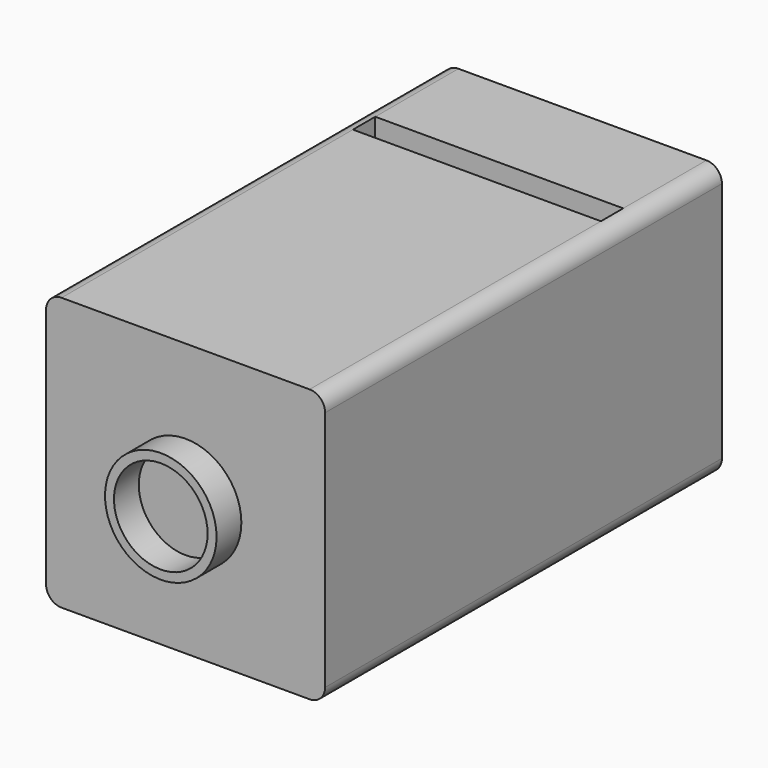
from build123d import *

# Parameters (mm, degrees)
F0_W     = 90
F0_H     = 160
F1_DEPTH = 88
F2_W     = 80
F2_H     = 9
F3_DEPTH = 12.5
F4_DEPTH = 50
F5_R     = 17.988747928
F6_DEPTH = 10
F7_R     = 15.1004844519
F8_DEPTH = 10
F9_R     = 4.99999


# Not quite as in the source:
# - a fillet or chamfer is up to 0.001 mm smaller than in the source, because OpenCascade refuses the exact size


with BuildPart() as f1:
    # F0 (on Top) → F1 (new body)
    with BuildSketch(Plane.XY):
        Rectangle(F0_W, F0_H)
    extrude(amount=F1_DEPTH)

    # F2 (on face) → F3 (cut, symmetric)
    with BuildSketch(Plane.XY.offset(88)):
        with Locations((0, 41.9618518679)):
            Rectangle(F2_W, F2_H)
    extrude(amount=F3_DEPTH, both=True, mode=Mode.SUBTRACT)

    # F4 (cut): a face of the model
    f4_faces = [f1.faces().sort_by_distance(p)[0] for p in [
        (0, 41.9618518679, 75.5),
    ]]
    extrude(f4_faces, amount=-F4_DEPTH, mode=Mode.SUBTRACT)

    # F5 (on face) → F6 (join)
    with BuildSketch(Plane.XZ.offset(80)):
        with Locations((0, 43)):
            Circle(F5_R)
    extrude(amount=F6_DEPTH)

    # F7 (on face) → F8 (cut)
    with BuildSketch(Plane.XZ.offset(90)):
        with Locations((0, 43)):
            Circle(F7_R)
    extrude(amount=-F8_DEPTH, mode=Mode.SUBTRACT)

    # F9 (radius 5 in the source; OpenCascade refuses exactly that, so slightly less here)
    f9_edges = [f1.edges().sort_by_distance(p)[0] for p in [
        (-45, 0, 88),
        (45, 0, 88),
        (45, 0, 0),
        (-45, 0, 0),
    ]]
    fillet(f9_edges, radius=F9_R)


solid = f1.part
